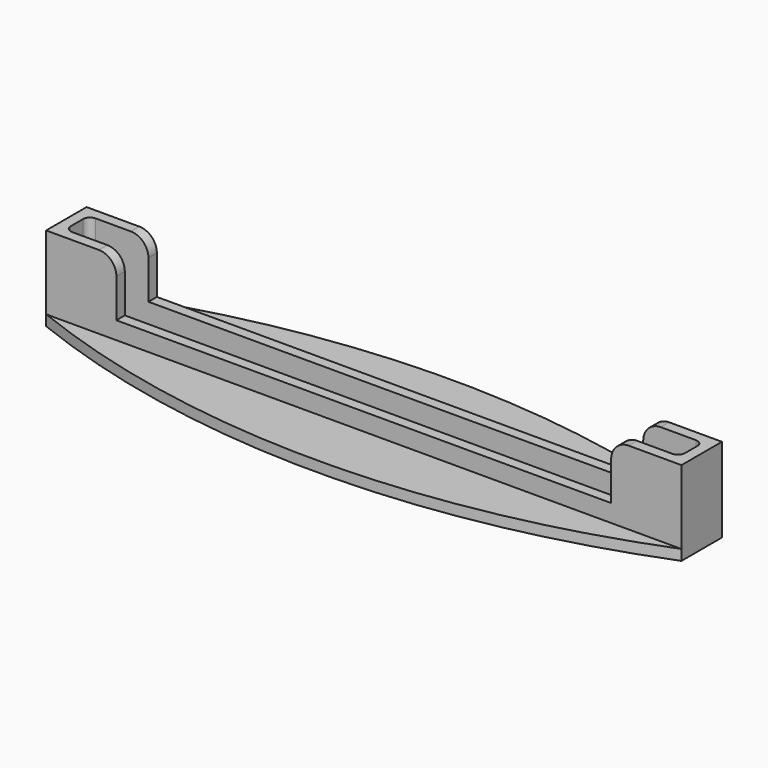
from build123d import *

# Parameters (mm, degrees)
F1_W        = 180.8
F1_H        = 14.4
F1_W_2      = 174.8
F1_H_2      = 8.4
F2_DEPTH    = 24
F3_T1_DEPTH = 24
F5_DEPTH    = 4.35
F6_W        = 140.8
F6_H        = 14.4
F7_DEPTH    = 16
F8_R        = 5
F10_DEPTH   = 3


# Not quite as in the source:
# - a fillet or chamfer that OpenCascade refuses, or shapes differently, is made with other operations: its cross-section is extruded or revolved along the edge and cut away or added
# - a pattern or mirror of a feature is missing from the dataset's text; its kind, count and spacing are read off the source's solid


with BuildPart() as f2:
    # F1 (on Top) → F2 (new body)
    with BuildSketch(Plane.XY):
        Rectangle(F1_W, F1_H)
        Rectangle(F1_W_2, F1_H_2, mode=Mode.SUBTRACT)
    extrude(amount=F2_DEPTH)

    # F3: fillet of radius 2 on 4 edges, made by hand

    # F3_s2 → F3_t1 (join)
    with BuildSketch(Plane.XY):
        with BuildLine():
            ThreePointArc((87.4004, -2.1990343146), (86.8142135624, -3.6142135624), (85.3990343146, -4.2004))
            Line((85.3990343146, -4.2004), (85.3990343146, -4.4005365685))
            ThreePointArc((85.3990343146, -4.4005365685), (86.3995171573, -4.4001365685), (87.4, -4.4001365685))
            Line((87.4, -4.4001365685), (87.6001365685, -4.2))
            ThreePointArc((87.6001365685, -4.2), (87.6001365685, -3.1995171573), (87.6005365685, -2.1990343146))
            Line((87.6005365685, -2.1990343146), (87.4004, -2.1990343146))
        make_face()
        with BuildLine():
            ThreePointArc((87.4004, 2.1990343146), (86.8142135624, 3.6142135624), (85.3990343146, 4.2004))
            Line((85.3990343146, 4.2004), (85.3990343146, 4.4005365685))
            ThreePointArc((85.3990343146, 4.4005365685), (86.3995171573, 4.4001365685), (87.4, 4.4001365685))
            Line((87.4, 4.4001365685), (87.6001365685, 4.2))
            ThreePointArc((87.6001365685, 4.2), (87.6001365685, 3.1995171573), (87.6005365685, 2.1990343146))
            Line((87.6005365685, 2.1990343146), (87.4004, 2.1990343146))
        make_face()
        with BuildLine():
            ThreePointArc((-85.3990343146, -4.2004), (-86.8142135624, -3.6142135624), (-87.4004, -2.1990343146))
            Line((-87.4004, -2.1990343146), (-87.6005365685, -2.1990343146))
            ThreePointArc((-87.6005365685, -2.1990343146), (-87.6001365685, -3.1995171573), (-87.6001365685, -4.2))
            Line((-87.6001365685, -4.2), (-87.4, -4.4001365685))
            ThreePointArc((-87.4, -4.4001365685), (-86.3995171573, -4.4001365685), (-85.3990343146, -4.4005365685))
            Line((-85.3990343146, -4.4005365685), (-85.3990343146, -4.2004))
        make_face()
        with BuildLine():
            ThreePointArc((-87.4004, 2.1990343146), (-86.8142135624, 3.6142135624), (-85.3990343146, 4.2004))
            Line((-85.3990343146, 4.2004), (-85.3990343146, 4.4005365685))
            ThreePointArc((-85.3990343146, 4.4005365685), (-86.3995171573, 4.4001365685), (-87.4, 4.4001365685))
            Line((-87.4, 4.4001365685), (-87.6001365685, 4.2))
            ThreePointArc((-87.6001365685, 4.2), (-87.6001365685, 3.1995171573), (-87.6005365685, 2.1990343146))
            Line((-87.6005365685, 2.1990343146), (-87.4004, 2.1990343146))
        make_face()
    extrude(amount=F3_T1_DEPTH)

    # F4 (on Front) → F5 (join, symmetric)
    with BuildSketch(Plane.XZ):
        with BuildLine():
            ThreePointArc((87.4, 8.75), (85.0568542495, 3.0931457505), (79.4, 0.75))
            Line((79.4, 0.75), (79.4, 0))
            Line((79.4, 0), (90.4, 0))
            Line((90.4, 0), (90.4, 8.75))
            Line((90.4, 8.75), (87.4, 8.75))
        make_face()
    f5 = extrude(amount=F5_DEPTH, both=True)

    # F5_copies: F5 across plane
    add(f5.mirror(Plane(origin=(0, 0, 0), x_dir=(0, 0, -1), z_dir=(-1, 0, 0))))

    # F6 (on face) → F7 (cut)
    with BuildSketch(Plane.XY.offset(24)):
        Rectangle(F6_W, F6_H)
    extrude(amount=-F7_DEPTH, mode=Mode.SUBTRACT)

    # F8
    f8_edges = [f2.edges().sort_by_distance(p)[0] for p in [
        (-70.4, 5.7, 24),
        (-70.4, -5.7, 24),
        (70.4, 5.7, 24),
        (70.4, -5.7, 24),
    ]]
    fillet(f8_edges, radius=F8_R)

    # F9 (on Top) → F10 (join)
    with BuildSketch(Plane.XY):
        with BuildLine():
            Line((90.4, -7.2), (-90.4, -7.2))
            ThreePointArc((-90.4, -7.2), (0, -24.4878132379), (90.4, -7.2))
        make_face()
        with BuildLine():
            Line((-90.4, 7.2), (90.4, 7.2))
            ThreePointArc((90.4, 7.2), (0, 24.4878132379), (-90.4, 7.2))
        make_face()
    extrude(amount=F10_DEPTH)


solid = f2.part
